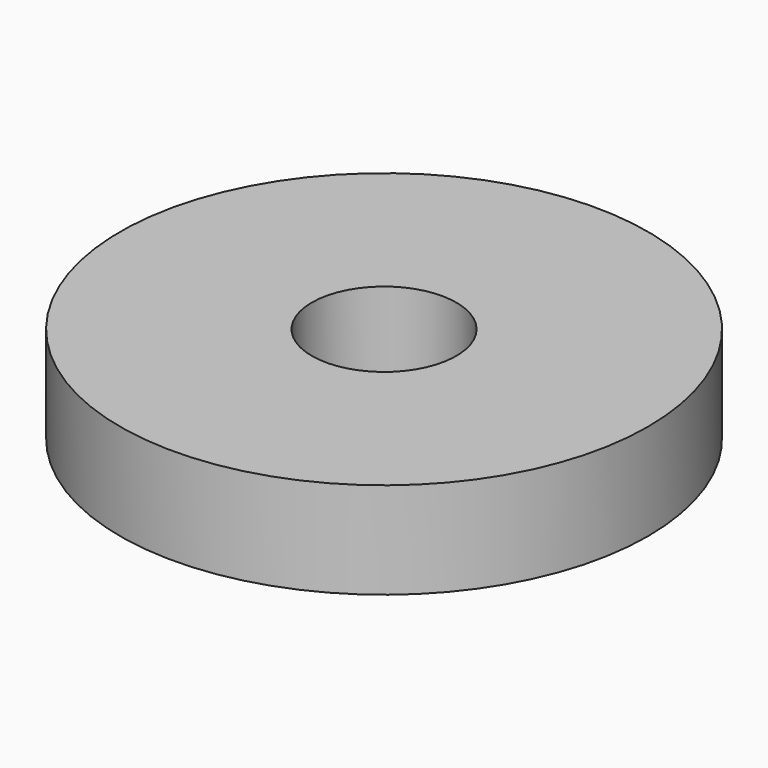
from build123d import *

# Parameters (mm, degrees)
F0_R     = 34.7832495942
F1_DEPTH = 12.7
F2_D     = 19.05


# Not quite as in the source:
# - a feature of the source that left no trace in its solid (it failed there, or was rolled back) is left out


with BuildPart() as f1:
    # F0 (on Top) → F1 (new body)
    with BuildSketch(Plane.XY):
        with Locations((-28.1662195921, -50.2411574125)):
            Circle(F0_R)
    extrude(amount=F1_DEPTH)

    # F2 (through all)
    with Locations(Plane(origin=(0, 0, 0), x_dir=(1, 0, 0), z_dir=(0, 0, -1))):
        with Locations((-28.1662195921, 50.2411574125)):
            Hole(F2_D / 2)


solid = f1.part
